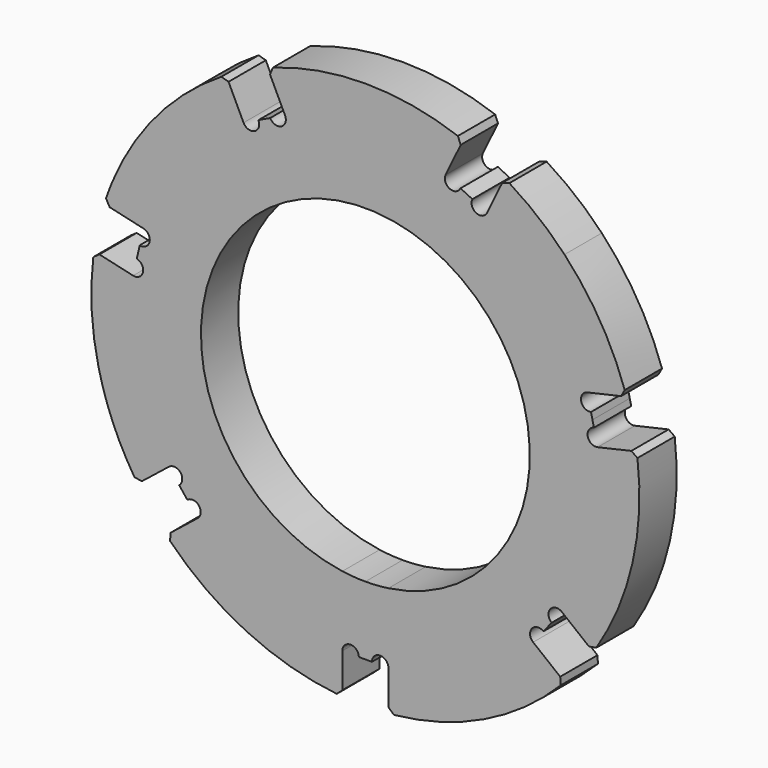
from build123d import *

# Parameters (mm, degrees)
F1_DEPTH    = 17
F2_DEPTH    = 17
F3_T1_DEPTH = 27.4714321234
F4_R        = 3
F5_DEPTH    = 25


# Not quite as in the source:
# - a fillet or chamfer that OpenCascade refuses, or shapes differently, is made with other operations: its cross-section is extruded or revolved along the edge and cut away or added


with BuildPart() as f1:
    # F0 (on Front) → F1 (new body)
    with BuildSketch(Plane.XZ):
        with BuildLine():
            Line((8.4, -85), (8.4, -99.6465754555))
            ThreePointArc((8.4, -99.6465754555), (43.3883739118, -90.0968867902), (72.6695154756, -68.6960080394))
            Line((72.6695154756, -68.6960080394), (61.2183616742, -59.5640176107))
            Line((61.2183616742, -59.5640176107), (66.4556760098, -52.996633158))
            Line((66.4556760098, -52.996633158), (71.6929903454, -46.4292487053))
            Line((71.6929903454, -46.4292487053), (83.1441441468, -55.5612391339))
            ThreePointArc((83.1441441468, -55.5612391339), (97.4927912182, -22.2520933956), (99.0174036101, 13.9840545736))
            Line((99.0174036101, 13.9840545736), (84.7380483807, 10.724884924))
            Line((84.7380483807, 10.724884924), (82.8688725355, 18.9142793863))
            Line((82.8688725355, 18.9142793863), (80.9996966902, 27.1036738486))
            Line((80.9996966902, 27.1036738486), (95.2790519196, 30.3628434982))
            ThreePointArc((95.2790519196, 30.3628434982), (86.1338388699, 50.8031672393), (72.6695154756, 68.6960080394))
            ThreePointArc((72.6695154756, 68.6960080394), (62.3489801859, 78.1831482468), (50.8031672393, 86.1338388699))
            Line((50.8031672393, 86.1338388699), (44.4482563154, 72.9377303631))
            Line((44.4482563154, 72.9377303631), (36.880117825, 76.5823537717))
            Line((36.880117825, 76.5823537717), (29.3119793346, 80.2269771803))
            Line((29.3119793346, 80.2269771803), (35.6668902585, 93.423085687))
            ThreePointArc((35.6668902585, 93.423085687), (0, 100), (-35.6668902585, 93.423085687))
            Line((-35.6668902585, 93.423085687), (-29.3119793346, 80.2269771803))
            Line((-29.3119793346, 80.2269771803), (-36.880117825, 76.5823537717))
            Line((-36.880117825, 76.5823537717), (-44.4482563154, 72.9377303631))
            Line((-44.4482563154, 72.9377303631), (-50.8031672393, 86.1338388699))
            ThreePointArc((-50.8031672393, 86.1338388699), (-75.3071466004, 65.793872594), (-92.1737821607, 38.7813599839))
            ThreePointArc((-92.1737821607, 38.7813599839), (-93.8208884318, 34.6069486355), (-95.2790519196, 30.3628434982))
            Line((-95.2790519196, 30.3628434982), (-80.9996966902, 27.1036738486))
            Line((-80.9996966902, 27.1036738486), (-82.8688725355, 18.9142793863))
            Line((-82.8688725355, 18.9142793863), (-84.7380483807, 10.724884924))
            Line((-84.7380483807, 10.724884924), (-99.0174036101, 13.9840545736))
            ThreePointArc((-99.0174036101, 13.9840545736), (-99.8993066541, -4.4864830351), (-97.3652676662, -22.8036105101))
            ThreePointArc((-97.3652676662, -22.8036105101), (-95.1056516295, -30.9016994375), (-92.1737821607, -38.7813599839))
            ThreePointArc((-92.1737821607, -38.7813599839), (-88.0595531857, -47.3868662473), (-83.1441441468, -55.5612391339))
            Line((-83.1441441468, -55.5612391339), (-71.6929903454, -46.4292487053))
            Line((-71.6929903454, -46.4292487053), (-66.4556760098, -52.996633158))
            Line((-66.4556760098, -52.996633158), (-61.2183616742, -59.5640176107))
            Line((-61.2183616742, -59.5640176107), (-72.6695154756, -68.6960080394))
            ThreePointArc((-72.6695154756, -68.6960080394), (-43.3883739118, -90.0968867902), (-8.4, -99.6465754555))
            Line((-8.4, -99.6465754555), (-8.4, -85))
            Line((-8.4, -85), (0, -85))
            Line((0, -85), (8.4, -85))
        make_face()
        with BuildLine():
            ThreePointArc((-8.4, -59.4090902135), (-39.3446311458, 45.2990066116), (60, 0))
            ThreePointArc((60, 0), (45.2990066116, -39.3446311458), (8.4, -59.4090902135))
            ThreePointArc((8.4, -59.4090902135), (4.2103792696, -59.8520902426), (0, -60))
            ThreePointArc((0, -60), (-4.2103792696, -59.8520902426), (-8.4, -59.4090902135))
        make_face(mode=Mode.SUBTRACT)
    extrude(amount=F1_DEPTH)

    # F0 (on Front) → F2 (join)
    with BuildSketch(Plane.XZ):
        with BuildLine():
            Line((8.4, -85), (8.4, -99.6465754555))
            ThreePointArc((8.4, -99.6465754555), (43.3883739118, -90.0968867902), (72.6695154756, -68.6960080394))
            Line((72.6695154756, -68.6960080394), (61.2183616742, -59.5640176107))
            Line((61.2183616742, -59.5640176107), (66.4556760098, -52.996633158))
            Line((66.4556760098, -52.996633158), (71.6929903454, -46.4292487053))
            Line((71.6929903454, -46.4292487053), (83.1441441468, -55.5612391339))
            ThreePointArc((83.1441441468, -55.5612391339), (97.4927912182, -22.2520933956), (99.0174036101, 13.9840545736))
            Line((99.0174036101, 13.9840545736), (84.7380483807, 10.724884924))
            Line((84.7380483807, 10.724884924), (82.8688725355, 18.9142793863))
            Line((82.8688725355, 18.9142793863), (80.9996966902, 27.1036738486))
            Line((80.9996966902, 27.1036738486), (95.2790519196, 30.3628434982))
            ThreePointArc((95.2790519196, 30.3628434982), (86.1338388699, 50.8031672393), (72.6695154756, 68.6960080394))
            ThreePointArc((72.6695154756, 68.6960080394), (62.3489801859, 78.1831482468), (50.8031672393, 86.1338388699))
            Line((50.8031672393, 86.1338388699), (44.4482563154, 72.9377303631))
            Line((44.4482563154, 72.9377303631), (36.880117825, 76.5823537717))
            Line((36.880117825, 76.5823537717), (29.3119793346, 80.2269771803))
            Line((29.3119793346, 80.2269771803), (35.6668902585, 93.423085687))
            ThreePointArc((35.6668902585, 93.423085687), (0, 100), (-35.6668902585, 93.423085687))
            Line((-35.6668902585, 93.423085687), (-29.3119793346, 80.2269771803))
            Line((-29.3119793346, 80.2269771803), (-36.880117825, 76.5823537717))
            Line((-36.880117825, 76.5823537717), (-44.4482563154, 72.9377303631))
            Line((-44.4482563154, 72.9377303631), (-50.8031672393, 86.1338388699))
            ThreePointArc((-50.8031672393, 86.1338388699), (-75.3071466004, 65.793872594), (-92.1737821607, 38.7813599839))
            ThreePointArc((-92.1737821607, 38.7813599839), (-93.8208884318, 34.6069486355), (-95.2790519196, 30.3628434982))
            Line((-95.2790519196, 30.3628434982), (-80.9996966902, 27.1036738486))
            Line((-80.9996966902, 27.1036738486), (-82.8688725355, 18.9142793863))
            Line((-82.8688725355, 18.9142793863), (-84.7380483807, 10.724884924))
            Line((-84.7380483807, 10.724884924), (-99.0174036101, 13.9840545736))
            ThreePointArc((-99.0174036101, 13.9840545736), (-99.8993066541, -4.4864830351), (-97.3652676662, -22.8036105101))
            ThreePointArc((-97.3652676662, -22.8036105101), (-95.1056516295, -30.9016994375), (-92.1737821607, -38.7813599839))
            ThreePointArc((-92.1737821607, -38.7813599839), (-88.0595531857, -47.3868662473), (-83.1441441468, -55.5612391339))
            Line((-83.1441441468, -55.5612391339), (-71.6929903454, -46.4292487053))
            Line((-71.6929903454, -46.4292487053), (-66.4556760098, -52.996633158))
            Line((-66.4556760098, -52.996633158), (-61.2183616742, -59.5640176107))
            Line((-61.2183616742, -59.5640176107), (-72.6695154756, -68.6960080394))
            ThreePointArc((-72.6695154756, -68.6960080394), (-43.3883739118, -90.0968867902), (-8.4, -99.6465754555))
            Line((-8.4, -99.6465754555), (-8.4, -85))
            Line((-8.4, -85), (0, -85))
            Line((0, -85), (8.4, -85))
        make_face()
        with BuildLine():
            ThreePointArc((-8.4, -59.4090902135), (-39.3446311458, 45.2990066116), (60, 0))
            ThreePointArc((60, 0), (45.2990066116, -39.3446311458), (8.4, -59.4090902135))
            ThreePointArc((8.4, -59.4090902135), (4.2103792696, -59.8520902426), (0, -60))
            ThreePointArc((0, -60), (-4.2103792696, -59.8520902426), (-8.4, -59.4090902135))
        make_face(mode=Mode.SUBTRACT)
    extrude(amount=F2_DEPTH)

    # F3: chamfer of 2 on 14 edges, made by hand

    # F3_s2 → F3_t1 (cut)
    with BuildSketch(Plane.XZ.offset(-5.2357160617)):
        with BuildLine():
            Line((-49.8497245383, 84.2910026161), (-52.6258418308, 85.1023869989))
            Line((-52.6258418308, 85.1023869989), (-52.6468614525, 85.1364189765))
            ThreePointArc((-52.6468614525, 85.1364189765), (-51.7226459051, 85.6315917204), (-50.8234885061, 86.1682924054))
            Line((-50.8234885061, 86.1682924054), (-50.7671284845, 86.1511942194))
            ThreePointArc((-50.7671284845, 86.1511942194), (-50.3171864094, 85.2168798732), (-49.8136857836, 84.3083579657))
            Line((-49.8136857836, 84.3083579657), (-49.8497245383, 84.2910026161))
        make_face()
        with BuildLine():
            Line((-33.7240496932, 94.2050103423), (-34.820564659, 91.528664556))
            Line((-34.820564659, 91.528664556), (-34.8566034137, 91.5113092064))
            ThreePointArc((-34.8566034137, 91.5113092064), (-35.2529869381, 92.4714159913), (-35.7029290132, 93.4057303375))
            Line((-35.7029290132, 93.4057303375), (-35.6811570146, 93.4604549213))
            ThreePointArc((-35.6811570146, 93.4604549213), (-34.7009320539, 93.8288170798), (-33.7375514449, 94.2426627353))
            Line((-33.7375514449, 94.2426627353), (-33.7240496932, 94.2050103423))
        make_face()
        with BuildLine():
            Line((34.820564659, 91.528664556), (33.7240496932, 94.2050103423))
            Line((33.7240496932, 94.2050103423), (33.7375514449, 94.2426627353))
            ThreePointArc((33.7375514449, 94.2426627353), (34.7009320539, 93.8288170798), (35.6811570146, 93.4604549213))
            Line((35.6811570146, 93.4604549213), (35.7029290132, 93.4057303375))
            ThreePointArc((35.7029290132, 93.4057303375), (35.2529869381, 92.4714159913), (34.8566034137, 91.5113092064))
            Line((34.8566034137, 91.5113092064), (34.820564659, 91.528664556))
        make_face()
        with BuildLine():
            Line((52.6258418308, 85.1023869989), (49.8497245383, 84.2910026161))
            Line((49.8497245383, 84.2910026161), (49.8136857836, 84.3083579657))
            ThreePointArc((49.8136857836, 84.3083579657), (50.3171864094, 85.2168798732), (50.7671284845, 86.1511942194))
            Line((50.7671284845, 86.1511942194), (50.8234885061, 86.1682924054))
            ThreePointArc((50.8234885061, 86.1682924054), (51.7226459051, 85.6315917204), (52.6468614525, 85.1364189765))
            Line((52.6468614525, 85.1364189765), (52.6258418308, 85.1023869989))
        make_face()
        with BuildLine():
            Line((93.270258458, 29.8433752407), (94.679043953, 32.369339466))
            Line((94.679043953, 32.369339466), (94.7168999837, 32.3822592545))
            ThreePointArc((94.7168999837, 32.3822592545), (94.9940004063, 31.371029419), (95.3171635404, 30.3749886356))
            Line((95.3171635404, 30.3749886356), (95.287952757, 30.3238463817))
            ThreePointArc((95.287952757, 30.3238463817), (94.2769420913, 30.0930897948), (93.2791592954, 29.8043781242))
            Line((93.2791592954, 29.8043781242), (93.270258458, 29.8433752407))
        make_face()
        with BuildLine():
            Line((99.3474010846, 11.915930473), (96.9821544092, 13.5804964832))
            Line((96.9821544092, 13.5804964832), (96.9732535718, 13.6194935997))
            ThreePointArc((96.9732535718, 13.6194935997), (97.9974921071, 13.7922951031), (99.0085027727, 14.0230516901))
            Line((99.0085027727, 14.0230516901), (99.0570105715, 13.9896481954))
            ThreePointArc((99.0570105715, 13.9896481954), (99.1980165479, 12.9520312295), (99.387113876, 11.9207152619))
            Line((99.387113876, 11.9207152619), (99.3474010846, 11.915930473))
        make_face()
        with BuildLine():
            Line((81.4855452716, -54.3145843248), (84.3387870156, -53.8411042425))
            Line((84.3387870156, -53.8411042425), (84.3724909621, -53.8626459227))
            ThreePointArc((84.3724909621, -53.8626459227), (83.7546489283, -54.7097832467), (83.1774018045, -55.5834636295))
            Line((83.1774018045, -55.5834636295), (83.1192045547, -55.5925123932))
            ThreePointArc((83.1192045547, -55.5925123932), (82.3084369507, -54.9459468044), (81.4606056795, -54.3458575841))
            Line((81.4606056795, -54.3458575841), (81.4855452716, -54.3145843248))
        make_face()
        with BuildLine():
            Line((71.2583410041, -70.2434647398), (71.0850439345, -67.3564004932))
            Line((71.0850439345, -67.3564004932), (71.1099835266, -67.3251272339))
            ThreePointArc((71.1099835266, -67.3251272339), (71.8836874636, -68.0181691912), (72.6944550677, -68.6647347801))
            Line((72.6944550677, -68.6647347801), (72.6985832818, -68.7234864426))
            ThreePointArc((72.6985832818, -68.7234864426), (71.9752574593, -69.4806729506), (71.2868424232, -70.2715301832))
            Line((71.2868424232, -70.2715301832), (71.2583410041, -70.2434647398))
        make_face()
        with BuildLine():
            Line((8.3405544935, -97.5725540781), (10.4897032578, -99.5080982979))
            Line((10.4897032578, -99.5080982979), (10.4938753609, -99.5478801224))
            ThreePointArc((10.4938753609, -99.5478801224), (9.4463385238, -99.5930132514), (8.40336, -99.6864340856))
            Line((8.40336, -99.6864340856), (8.36, -99.6465754555))
            ThreePointArc((8.36, -99.6465754555), (8.36, -98.6095647668), (8.3005544935, -97.5725540781))
            Line((8.3005544935, -97.5725540781), (8.3405544935, -97.5725540781))
        make_face()
        with BuildLine():
            Line((-10.4897032578, -99.5080982979), (-8.3405544935, -97.5725540781))
            Line((-8.3405544935, -97.5725540781), (-8.3005544935, -97.5725540781))
            ThreePointArc((-8.3005544935, -97.5725540781), (-8.36, -98.6095647668), (-8.36, -99.6465754555))
            Line((-8.36, -99.6465754555), (-8.40336, -99.6864340856))
            ThreePointArc((-8.40336, -99.6864340856), (-9.4463385238, -99.5930132514), (-10.4938753609, -99.5478801224))
            Line((-10.4938753609, -99.5478801224), (-10.4897032578, -99.5080982979))
        make_face()
        with BuildLine():
            Line((-71.0850439345, -67.3564004932), (-71.2583410041, -70.2434647398))
            Line((-71.2583410041, -70.2434647398), (-71.2868424232, -70.2715301832))
            ThreePointArc((-71.2868424232, -70.2715301832), (-71.9752574593, -69.4806729506), (-72.6985832818, -68.7234864426))
            Line((-72.6985832818, -68.7234864426), (-72.6944550677, -68.6647347801))
            ThreePointArc((-72.6944550677, -68.6647347801), (-71.8836874636, -68.0181691912), (-71.1099835266, -67.3251272339))
            Line((-71.1099835266, -67.3251272339), (-71.0850439345, -67.3564004932))
        make_face()
        with BuildLine():
            Line((-84.3387870156, -53.8411042425), (-81.4855452716, -54.3145843248))
            Line((-81.4855452716, -54.3145843248), (-81.4606056795, -54.3458575841))
            ThreePointArc((-81.4606056795, -54.3458575841), (-82.3084369507, -54.9459468044), (-83.1192045547, -55.5925123932))
            Line((-83.1192045547, -55.5925123932), (-83.1774018045, -55.5834636295))
            ThreePointArc((-83.1774018045, -55.5834636295), (-83.7546489283, -54.7097832467), (-84.3724909621, -53.8626459227))
            Line((-84.3724909621, -53.8626459227), (-84.3387870156, -53.8411042425))
        make_face()
        with BuildLine():
            Line((-94.679043953, 32.369339466), (-93.270258458, 29.8433752407))
            Line((-93.270258458, 29.8433752407), (-93.2791592954, 29.8043781242))
            ThreePointArc((-93.2791592954, 29.8043781242), (-94.2769420913, 30.0930897948), (-95.287952757, 30.3238463817))
            Line((-95.287952757, 30.3238463817), (-95.3171635404, 30.3749886356))
            ThreePointArc((-95.3171635404, 30.3749886356), (-94.9940004063, 31.371029419), (-94.7168999837, 32.3822592545))
            Line((-94.7168999837, 32.3822592545), (-94.679043953, 32.369339466))
        make_face()
        with BuildLine():
            Line((-99.3474010846, 11.915930473), (-96.9821544092, 13.5804964832))
            Line((-96.9821544092, 13.5804964832), (-96.9732535718, 13.6194935997))
            ThreePointArc((-96.9732535718, 13.6194935997), (-97.9974921071, 13.7922951031), (-99.0085027727, 14.0230516901))
            Line((-99.0085027727, 14.0230516901), (-99.0570105715, 13.9896481954))
            ThreePointArc((-99.0570105715, 13.9896481954), (-99.1980165479, 12.9520312295), (-99.387113876, 11.9207152619))
            Line((-99.387113876, 11.9207152619), (-99.3474010846, 11.915930473))
        make_face()
    extrude(amount=F3_T1_DEPTH, mode=Mode.SUBTRACT)

    # F4 (on face) → F5 (cut)
    with BuildSketch(Plane.XZ.offset(17)):
        with BuildLine():
            ThreePointArc((-39.042443108, 75.5410327978), (-43.047000929, 76.9422881842), (-44.4482563154, 72.9377303631))
            Line((-44.4482563154, 72.9377303631), (-39.042443108, 75.5410327978))
        make_face()
        with BuildLine():
            Line((-39.042443108, 75.5410327978), (-44.4482563154, 72.9377303631))
            ThreePointArc((-44.4482563154, 72.9377303631), (-41.0777869098, 71.3145978439), (-38.7453497117, 74.2393815805))
            ThreePointArc((-38.7453497117, 74.2393815805), (-38.8205659751, 74.9069443823), (-39.042443108, 75.5410327978))
        make_face()
        with BuildLine():
            ThreePointArc((-29.3119793346, 80.2269771803), (-33.3165371557, 81.6282325666), (-34.717792542, 77.6236747456))
            Line((-34.717792542, 77.6236747456), (-29.3119793346, 80.2269771803))
        make_face()
        with BuildLine():
            Line((-29.3119793346, 80.2269771803), (-34.717792542, 77.6236747456))
            ThreePointArc((-34.717792542, 77.6236747456), (-31.3473231365, 76.0005422264), (-29.0148859383, 78.9253259629))
            ThreePointArc((-29.0148859383, 78.9253259629), (-29.0901022018, 79.5928887648), (-29.3119793346, 80.2269771803))
        make_face()
        with Locations((-84.0704855788, 13.6496686605)):
            Circle(F4_R)
        with Locations((-81.6672594921, 24.1788901121)):
            Circle(F4_R)
        with Locations((-63.0888310797, -57.2185231633)):
            Circle(F4_R)
        with Locations((-69.8225209398, -48.7747431527)):
            Circle(F4_R)
        with Locations((5.4, -85)):
            Circle(F4_R)
        with Locations((-5.4, -85)):
            Circle(F4_R)
        with Locations((69.8225209398, -48.7747431527)):
            Circle(F4_R)
        with Locations((63.0888310797, -57.2185231633)):
            Circle(F4_R)
        with Locations((81.6672594921, 24.1788901121)):
            Circle(F4_R)
        with Locations((84.0704855788, 13.6496686605)):
            Circle(F4_R)
        with Locations((32.0148859383, 78.9253259629)):
            Circle(F4_R)
        with Locations((41.7453497117, 74.2393815805)):
            Circle(F4_R)
    extrude(amount=-F5_DEPTH, mode=Mode.SUBTRACT)


solid = f1.part
